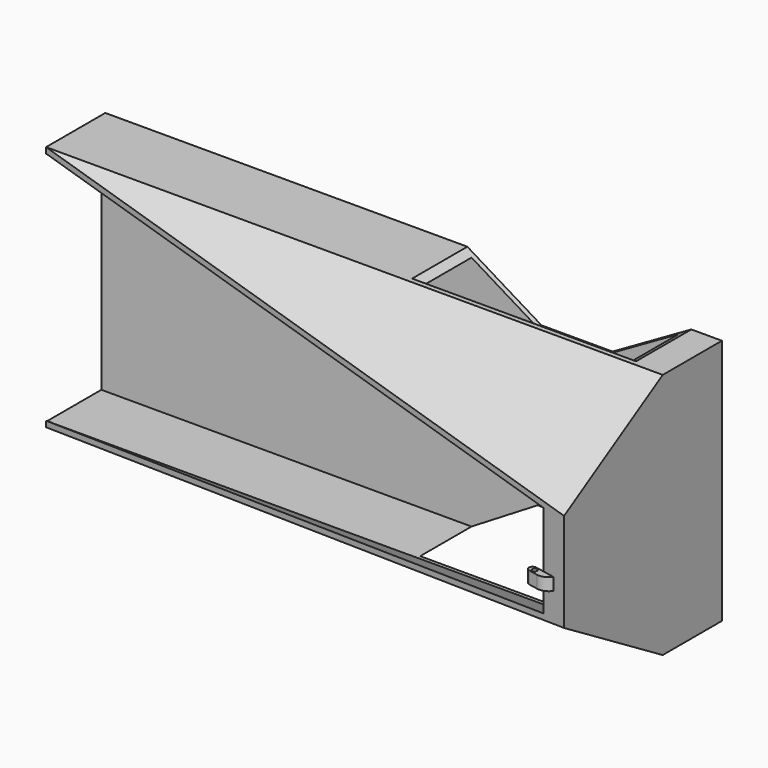
from build123d import *

# Parameters (mm, degrees)
F1_DEPTH     = 5
F3_DEPTH     = 25
F5_DEPTH     = 2
F7_DEPTH     = 250
F9_DEPTH     = 248
F11_DEPTH    = 110
F13_W        = 5
F13_H        = 5
F14_DEPTH    = 3
F15_T1_DEPTH = 27.9128784748
F16_DEPTH    = 5
F18_D        = 2
F19_R        = 1.49999


# Not quite as in the source:
# - a fillet or chamfer that OpenCascade refuses, or shapes differently, is made with other operations: its cross-section is extruded or revolved along the edge and cut away or added
# - a fillet or chamfer is up to 0.001 mm smaller than in the source, because OpenCascade refuses the exact size


with BuildPart() as f1:
    # F0 (on Front) → F1 (new body)
    with BuildSketch(Plane.XZ):
        Polygon((20.074704662, 60.7631485909), (-126.7197424916, 60.7631485909), (-126.7197424916, 10.7631485909), (-126.7197424916, -39.2368514091), (20.074704662, -39.2368514091), (50.1353926957, -20.9532961249), (78.9564624429, -20.9532961249), (110.8765751123, -39.2368514091), (123.2802575084, -39.2368514091), (123.2802575084, 10.7631485909), (123.2802575084, 60.7631485909), (110.8765751123, 60.7631485909), (78.9564624429, 42.4795933068), (50.1353926957, 42.4795933068), align=None)
    extrude(amount=F1_DEPTH)

    # F2 (on face) → F3 (join)
    with BuildSketch(Plane.XZ.offset(5)):
        Polygon((-126.7197424916, -39.2368514091), (20.074704662, -39.2368514091), (50.1353926957, -20.9532961249), (78.9564624429, -20.9532961249), (110.8765751123, -39.2368514091), (123.2802575084, -39.2368514091), (123.2802575084, 60.7631485909), (110.8765751123, 60.7631485909), (78.9564624429, 42.4795933068), (50.1353926957, 42.4795933068), (20.074704662, 60.7631485909), (-126.7197424916, 60.7631485909), align=None)
        Polygon((49.574933962, -18.9532961249), (19.5142459283, -37.2368514091), (-124.7197424916, -37.2368514091), (-124.7197424916, 58.7631485909), (19.5142459283, 58.7631485909), (49.574933962, 40.4795933068), (79.4886903674, 40.4795933068), (111.4088030368, 58.7631485909), (121.2802575084, 58.7631485909), (121.2802575084, -37.2368514091), (111.4088030368, -37.2368514091), (79.4886903674, -18.9532961249), align=None, mode=Mode.SUBTRACT)
    extrude(amount=F3_DEPTH)

    # F4 (on face) → F5 (join)
    with BuildSketch(Plane.XZ.offset(30)):
        Polygon((110.8765751123, 60.7631485909), (20.074704662, 60.7631485909), (50.1353926957, 42.4795933068), (78.9564624429, 42.4795933068), align=None)
        Polygon((50.1353926957, -20.9532961249), (20.074704662, -39.2368514091), (110.8765751123, -39.2368514091), (78.9564624429, -20.9532961249), align=None)
    extrude(amount=-F5_DEPTH)

    # F6 (on face) → F7 (join)
    with BuildSketch(Plane.YZ.offset(123.2802575084)):
        Polygon((-80, -9.2368514091), (-30, -39.2368514091), (-30, 60.7631485909), (-80, 30.7631485909), align=None)
    extrude(amount=-F7_DEPTH)

    # F8 (on face) → F9 (cut)
    with BuildSketch(Plane(origin=(-126.7197424916, 0, 0), x_dir=(0, -1, 0), z_dir=(-1, 0, 0))):
        Polygon((78, 29.630767833), (29.4460320701, 58.7631485909), (2, 58.7631485909), (2, -37.2368514091), (29.4460320701, -37.2368514091), (78, -8.1044706511), align=None)
    extrude(amount=-F9_DEPTH, mode=Mode.SUBTRACT)

    # F10 (on face) → F11 (cut)
    with BuildSketch(Plane(origin=(0, 0, -39.2368514091), x_dir=(1, 0, 0), z_dir=(0, 0, -1))):
        Polygon((-126.7197424916, 80), (-126.7197424916, 30), (123.2802575084, 80), align=None)
    extrude(amount=-F11_DEPTH, mode=Mode.SUBTRACT)

    # F13 (on face) → F14 (join)
    with BuildSketch(Plane(origin=(-10.6430670189, -53.2153350945, 0), x_dir=(0.9805806757, -0.1961161351, 0), z_dir=(-0.1961161351, -0.9805806757, 0))):
        with Locations((128.8774899908, 4.3955293489)):
            Rectangle(F13_W, F13_H)
    extrude(amount=F14_DEPTH)

    # F15: fillet of radius 5 on 1 edges, made by hand

    # F15_s2 → F15_t1 (cut)
    with BuildSketch(Plane.XY.offset(-9.5609098885)):
        with BuildLine():
            ThreePointArc((118.1831608869, -78.9805806757), (115.9468261093, -80.7598517163), (113.1012273101, -81.0236056685))
            Line((113.1012273101, -81.0236056685), (117.5948124814, -81.9223227028))
            Line((117.5948124814, -81.9223227028), (118.1831608869, -78.9805806757))
        make_face()
    extrude(amount=F15_T1_DEPTH, mode=Mode.SUBTRACT)

    # F16 (add): a face of the model
    f16_faces = [f1.faces().sort_by_distance(p)[0] for p in [
        (112.9860833057, -79.4708710135, 4.3955293489),
    ]]
    extrude(f16_faces, amount=F16_DEPTH)

    # F18 (through all)
    with Locations(Plane.XY.offset(6.8955293489)):
        with Locations((110.5346316165, -78.9805806757)):
            Hole(F18_D / 2)

    # F19 (radius 1.5 in the source; OpenCascade refuses exactly that, so slightly less here)
    f19_edges = [f1.edges().sort_by_distance(p)[0] for p in [
        (108.377354, -77.019419, 4.395529),
        (107.789006, -79.961161, 4.395529),
    ]]
    fillet(f19_edges, radius=F19_R)


solid = f1.part
